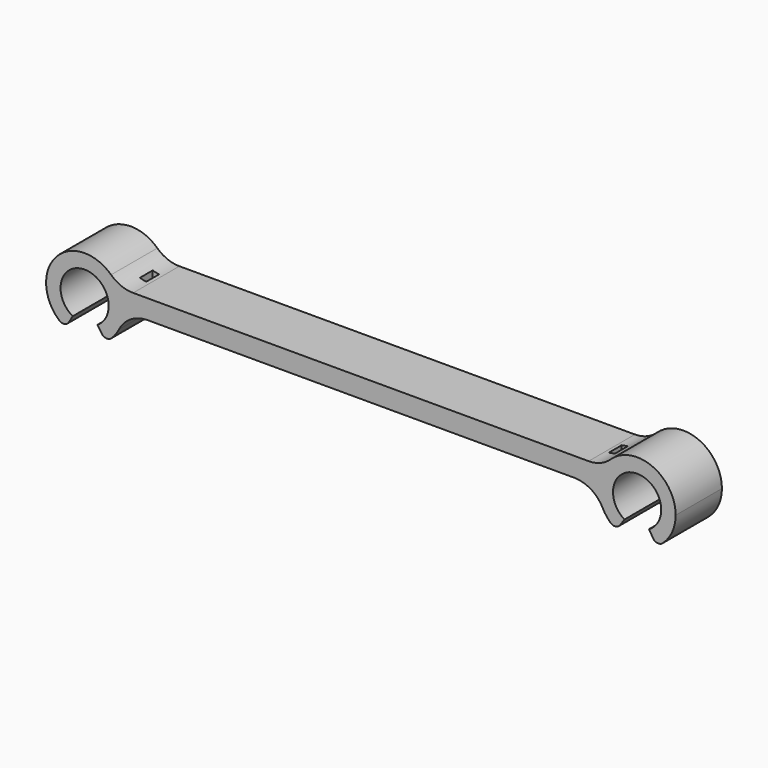
from build123d import *

# Parameters (mm, degrees)
F1_DEPTH      = 9
F2_R          = 1
F2_2_R        = 1
F3_W          = 86
F3_H          = 9
F4_DEPTH      = 3
F7_R          = 2
F8_DEPTH      = 25
F9_W          = 1
F9_H          = 2.5
F10_DEPTH     = 25
F11_R         = 3.75
F12_DEPTH     = 25
F13_T1_DEPTH  = 3.25
F13_T3_DEPTH  = 3.25
F13_T8_DEPTH  = 14.8842050314
F13_T13_DEPTH = 9
F13_T18_DEPTH = 9
F13_T23_DEPTH = 14.8842050314
F13_T28_DEPTH = 14.8842050314
F13_T33_DEPTH = 9
F13_T38_DEPTH = 9
F13_T43_DEPTH = 14.8842050314
F13_T48_DEPTH = 22.2397948557
F13_T54_DEPTH = 12.7448974278
F13_T60_DEPTH = 22.2397948557
F13_T66_DEPTH = 12.7448974278
F13_T72_DEPTH = 22.2397948557
F13_T78_DEPTH = 12.7448974278
F13_T84_DEPTH = 22.2397948557
F13_T90_DEPTH = 12.7448974278


# Not quite as in the source:
# - a fillet or chamfer that OpenCascade refuses, or shapes differently, is made with other operations: its cross-section is extruded or revolved along the edge and cut away or added
# - a feature names something its author has since deleted; it is built from what else it names


with BuildPart() as f1:
    # F0 (on Front) → F1 (new body)
    with BuildSketch(Plane.XZ):
        with BuildLine():
            ThreePointArc((-43.9727372119, -1.7475074582), (-44.0135397319, 1.7241627568), (-41, 0))
            Line((-41, 0), (-37, 0))
            ThreePointArc((-37, 0), (-46.0022354873, 5.1948611222), (-45.9955273596, -5.1987321375))
            Line((-45.9955273596, -5.1987321375), (-43.9727372119, -1.7475074582))
        make_face()
        with BuildLine():
            Line((-37, 0), (-41, 0))
            ThreePointArc((-41, 0), (-41.2758372432, -1.0135397319), (-42.0272627881, -1.7475074582))
            Line((-42.0272627881, -1.7475074582), (-39.7389427056, -5.0364179059))
            ThreePointArc((-39.7389427056, -5.0364179059), (-37.7290255281, -2.8665010233), (-37, 0))
        make_face()
    extrude(amount=F1_DEPTH)

    # F2
    f2_edges = [f1.edges().sort_by_distance(p)[0] for p in [
        (-42.027263, -4.5, -1.747507),
        (-43.972737, -4.5, -1.747507),
        (-39.738943, -4.5, -5.036418),
        (-45.995527, -4.5, -5.198732),
    ]]
    fillet(f2_edges, radius=F2_R)



with BuildPart() as f1b:
    # F0 (on Front) → F1, piece 2 (new body)
    with BuildSketch(Plane.XZ):
        with BuildLine():
            Line((41, 0), (37, 0))
            ThreePointArc((37, 0), (37.7290255281, -2.8665010233), (39.7389427056, -5.0364179059))
            Line((39.7389427056, -5.0364179059), (42.0272627881, -1.7475074582))
            ThreePointArc((42.0272627881, -1.7475074582), (41.2758372432, -1.0135397319), (41, 0))
        make_face()
        with BuildLine():
            ThreePointArc((49, 0), (43, 6), (37, 0))
            Line((37, 0), (41, 0))
            ThreePointArc((41, 0), (43, 2), (45, 0))
            ThreePointArc((45, 0), (44.7241627568, -1.0135397319), (43.9727372119, -1.7475074582))
            Line((43.9727372119, -1.7475074582), (45.9955273596, -5.1987321375))
            ThreePointArc((45.9955273596, -5.1987321375), (48.1948611222, -3.0022354873), (49, 0))
        make_face()
    extrude(amount=F1_DEPTH)

    # F2#2
    f2_2_edges = [f1b.edges().sort_by_distance(p)[0] for p in [
        (42.027263, -4.5, -1.747507),
        (43.972737, -4.5, -1.747507),
        (39.738943, -4.5, -5.036418),
        (45.995527, -4.5, -5.198732),
    ]]
    fillet(f2_2_edges, radius=F2_2_R)


with BuildPart() as f1_1:
    add(f1.part)

    add(f1b.part)  # F4 merges F1b
    # F3 (on Top) → F4 (join)
    with BuildSketch(Plane.XY):
        with Locations((0.0100198983, -4.5)):
            Rectangle(F3_W, F3_H)
    extrude(amount=F4_DEPTH)

    # F5: union 

    # F6: union 

    # F7 (on Front) → F8 (cut)
    with BuildSketch(Plane.XZ):
        with Locations((-43.0078394711, 0)):
            Circle(F7_R)
        with Locations((42.9660789669, 0)):
            Circle(F7_R)
    extrude(amount=F8_DEPTH, mode=Mode.SUBTRACT)

    # F9 (on face) → F10 (cut)
    with BuildSketch(Plane(origin=(0, 0, 0), x_dir=(1, 0, 0), z_dir=(0, 0, -1))):
        with Locations((36.5, 4.5)):
            Rectangle(F9_W, F9_H)
        with Locations((-36.5, 4.5)):
            Rectangle(F9_W, F9_H)
    extrude(amount=-F10_DEPTH, mode=Mode.SUBTRACT)

    # F11 (on Front) → F12 (cut)
    with BuildSketch(Plane.XZ):
        with Locations((-43, 0)):
            Circle(F11_R)
        with Locations((43, 0)):
            Circle(F11_R)
    extrude(amount=F12_DEPTH, mode=Mode.SUBTRACT)

    # F13: fillet of radius 5 on 6 edges, made by hand

    # F13_s2 → F13_t1 (join)
    with BuildSketch(Plane.XZ.offset(5.75)):
        with BuildLine():
            ThreePointArc((-37.655658743, -2.7272727273), (-35.8132058682, -0.7359856729), (-33.2020410289, 0))
            Line((-33.2020410289, 0), (-37, 0))
            ThreePointArc((-37, 0), (-37.1662170274, -1.4024892973), (-37.655658743, -2.7272727273))
        make_face()
        with BuildLine():
            ThreePointArc((37.655658743, -2.7272727273), (35.8132058682, -0.7359856729), (33.2020410289, 0))
            Line((33.2020410289, 0), (37, 0))
            ThreePointArc((37, 0), (37.1662170274, -1.4024892973), (37.655658743, -2.7272727273))
        make_face()
    extrude(amount=F13_T1_DEPTH)

    # F13_s4 → F13_t3 (join)
    with BuildSketch(Plane.XZ):
        with BuildLine():
            ThreePointArc((37.655658743, -2.7272727273), (35.8132058682, -0.7359856729), (33.2020410289, 0))
            Line((33.2020410289, 0), (37, 0))
            ThreePointArc((37, 0), (37.1662170274, -1.4024892973), (37.655658743, -2.7272727273))
        make_face()
        with BuildLine():
            ThreePointArc((-37.655658743, -2.7272727273), (-35.8132058682, -0.7359856729), (-33.2020410289, 0))
            Line((-33.2020410289, 0), (-37, 0))
            ThreePointArc((-37, 0), (-37.1662170274, -1.4024892973), (-37.655658743, -2.7272727273))
        make_face()
    extrude(amount=F13_T3_DEPTH)


with BuildPart() as f13_tool6:
    # F13_s7 → F13_t8 (new body)
    with BuildSketch(Plane.XZ.offset(9)):
        with BuildLine():
            ThreePointArc((35.4501655647, 3), (37.2965379294, 3.3533981136), (38.8819084899, 4.3636363636))
            ThreePointArc((38.8819084899, 4.3636363636), (38.2932324209, 3.7210669111), (37.8038475773, 3))
            Line((37.8038475773, 3), (35.4501655647, 3))
        make_face()
    extrude(amount=-F13_T8_DEPTH)

    split(bisect_by=Plane.XZ.offset(5.75), keep=Keep.TOP)


with BuildPart() as f1_2:
    add(f1_1.part)

    # F13_t5: union F13_tool6
    add(f13_tool6.part)


with BuildPart() as f13_tool11:
    # F13_s12 → F13_t13 (new body)
    with BuildSketch(Plane.XZ.offset(9)):
        with BuildLine():
            ThreePointArc((35.4501655647, 3), (37.2965379294, 3.3533981136), (38.8819084899, 4.3636363636))
            ThreePointArc((38.8819084899, 4.3636363636), (38.2932324209, 3.7210669111), (37.8038475773, 3))
            Line((37.8038475773, 3), (35.4501655647, 3))
        make_face()
    extrude(amount=-F13_T13_DEPTH)

    split(bisect_by=Plane.YZ.offset(36), keep=Keep.BOTTOM)


with BuildPart() as f1_3:
    add(f1_2.part)

    # F13_t10: union F13_tool11
    add(f13_tool11.part)


with BuildPart() as f13_tool16:
    # F13_s17 → F13_t18 (new body)
    with BuildSketch(Plane.XZ.offset(9)):
        with BuildLine():
            ThreePointArc((35.4501655647, 3), (37.2965379294, 3.3533981136), (38.8819084899, 4.3636363636))
            ThreePointArc((38.8819084899, 4.3636363636), (38.2932324209, 3.7210669111), (37.8038475773, 3))
            Line((37.8038475773, 3), (35.4501655647, 3))
        make_face()
    extrude(amount=-F13_T18_DEPTH)

    split(bisect_by=Plane.YZ.offset(37), keep=Keep.TOP)


with BuildPart() as f1_4:
    add(f1_3.part)

    # F13_t15: union F13_tool16
    add(f13_tool16.part)


with BuildPart() as f13_tool21:
    # F13_s22 → F13_t23 (new body)
    with BuildSketch(Plane.XZ.offset(14.8842050314)):
        with BuildLine():
            ThreePointArc((35.4501655647, 3), (37.2965379294, 3.3533981136), (38.8819084899, 4.3636363636))
            ThreePointArc((38.8819084899, 4.3636363636), (38.2932324209, 3.7210669111), (37.8038475773, 3))
            Line((37.8038475773, 3), (35.4501655647, 3))
        make_face()
    extrude(amount=-F13_T23_DEPTH)

    split(bisect_by=Plane.XZ.offset(3.25), keep=Keep.BOTTOM)


with BuildPart() as f1_5:
    add(f1_4.part)

    # F13_t20: union F13_tool21
    add(f13_tool21.part)


with BuildPart() as f13_tool26:
    # F13_s27 → F13_t28 (new body)
    with BuildSketch(Plane.XZ.offset(9)):
        with BuildLine():
            ThreePointArc((-35.4501655647, 3), (-37.2965379294, 3.3533981136), (-38.8819084899, 4.3636363636))
            ThreePointArc((-38.8819084899, 4.3636363636), (-38.2932324209, 3.7210669111), (-37.8038475773, 3))
            Line((-37.8038475773, 3), (-35.4501655647, 3))
        make_face()
    extrude(amount=-F13_T28_DEPTH)

    split(bisect_by=Plane.XZ.offset(5.75), keep=Keep.TOP)


with BuildPart() as f1_6:
    add(f1_5.part)

    # F13_t25: union F13_tool26
    add(f13_tool26.part)


with BuildPart() as f13_tool31:
    # F13_s32 → F13_t33 (new body)
    with BuildSketch(Plane.XZ.offset(9)):
        with BuildLine():
            ThreePointArc((-35.4501655647, 3), (-37.2965379294, 3.3533981136), (-38.8819084899, 4.3636363636))
            ThreePointArc((-38.8819084899, 4.3636363636), (-38.2932324209, 3.7210669111), (-37.8038475773, 3))
            Line((-37.8038475773, 3), (-35.4501655647, 3))
        make_face()
    extrude(amount=-F13_T33_DEPTH)

    split(bisect_by=Plane.YZ.offset(-36), keep=Keep.TOP)


with BuildPart() as f1_7:
    add(f1_6.part)

    # F13_t30: union F13_tool31
    add(f13_tool31.part)


with BuildPart() as f13_tool36:
    # F13_s37 → F13_t38 (new body)
    with BuildSketch(Plane.XZ.offset(9)):
        with BuildLine():
            ThreePointArc((-35.4501655647, 3), (-37.2965379294, 3.3533981136), (-38.8819084899, 4.3636363636))
            ThreePointArc((-38.8819084899, 4.3636363636), (-38.2932324209, 3.7210669111), (-37.8038475773, 3))
            Line((-37.8038475773, 3), (-35.4501655647, 3))
        make_face()
    extrude(amount=-F13_T38_DEPTH)

    split(bisect_by=Plane.YZ.offset(-37), keep=Keep.BOTTOM)


with BuildPart() as f1_8:
    add(f1_7.part)

    # F13_t35: union F13_tool36
    add(f13_tool36.part)


with BuildPart() as f13_tool41:
    # F13_s42 → F13_t43 (new body)
    with BuildSketch(Plane.XZ.offset(14.8842050314)):
        with BuildLine():
            ThreePointArc((-35.4501655647, 3), (-37.2965379294, 3.3533981136), (-38.8819084899, 4.3636363636))
            ThreePointArc((-38.8819084899, 4.3636363636), (-38.2932324209, 3.7210669111), (-37.8038475773, 3))
            Line((-37.8038475773, 3), (-35.4501655647, 3))
        make_face()
    extrude(amount=-F13_T43_DEPTH)

    split(bisect_by=Plane.XZ.offset(3.25), keep=Keep.BOTTOM)


with BuildPart() as f1_9:
    add(f1_8.part)

    # F13_t40: union F13_tool41
    add(f13_tool41.part)


with BuildPart() as f13_tool46:
    # F13_s47 → F13_t48 (new body)
    with BuildSketch(Plane.XZ.offset(18.4948974278)):
        with BuildLine():
            ThreePointArc((-37.655658743, -2.7272727273), (-35.8132058682, -0.7359856729), (-33.2020410289, 0))
            Line((-33.2020410289, 0), (-37, 0))
            ThreePointArc((-37, 0), (-37.1662170274, -1.4024892973), (-37.655658743, -2.7272727273))
        make_face()
    extrude(amount=-F13_T48_DEPTH)

    split(bisect_by=Plane.XZ.offset(3.25), keep=Keep.BOTTOM)

    split(bisect_by=Plane.XZ, keep=Keep.TOP)


with BuildPart() as f1_10:
    add(f1_9.part)

    # F13_t45: union F13_tool46
    add(f13_tool46.part)


with BuildPart() as f13_tool52:
    # F13_s53 → F13_t54 (new body)
    with BuildSketch(Plane.XZ.offset(9)):
        with BuildLine():
            ThreePointArc((-37.655658743, -2.7272727273), (-35.8132058682, -0.7359856729), (-33.2020410289, 0))
            Line((-33.2020410289, 0), (-37, 0))
            ThreePointArc((-37, 0), (-37.1662170274, -1.4024892973), (-37.655658743, -2.7272727273))
        make_face()
    extrude(amount=-F13_T54_DEPTH)

    split(bisect_by=Plane.YZ.offset(-36), keep=Keep.TOP)

    split(bisect_by=Plane.XZ, keep=Keep.TOP)


with BuildPart() as f1_11:
    add(f1_10.part)

    # F13_t51: union F13_tool52
    add(f13_tool52.part)


with BuildPart() as f13_tool58:
    # F13_s59 → F13_t60 (new body)
    with BuildSketch(Plane.XZ.offset(18.4948974278)):
        with BuildLine():
            ThreePointArc((37.655658743, -2.7272727273), (35.8132058682, -0.7359856729), (33.2020410289, 0))
            Line((33.2020410289, 0), (37, 0))
            ThreePointArc((37, 0), (37.1662170274, -1.4024892973), (37.655658743, -2.7272727273))
        make_face()
    extrude(amount=-F13_T60_DEPTH)

    split(bisect_by=Plane.XZ.offset(3.25), keep=Keep.BOTTOM)

    split(bisect_by=Plane.XZ, keep=Keep.TOP)


with BuildPart() as f1_12:
    add(f1_11.part)

    # F13_t57: union F13_tool58
    add(f13_tool58.part)


with BuildPart() as f13_tool64:
    # F13_s65 → F13_t66 (new body)
    with BuildSketch(Plane.XZ.offset(9)):
        with BuildLine():
            ThreePointArc((37.655658743, -2.7272727273), (35.8132058682, -0.7359856729), (33.2020410289, 0))
            Line((33.2020410289, 0), (37, 0))
            ThreePointArc((37, 0), (37.1662170274, -1.4024892973), (37.655658743, -2.7272727273))
        make_face()
    extrude(amount=-F13_T66_DEPTH)

    split(bisect_by=Plane.YZ.offset(36), keep=Keep.BOTTOM)

    split(bisect_by=Plane.XZ, keep=Keep.TOP)


with BuildPart() as f1_13:
    add(f1_12.part)

    # F13_t63: union F13_tool64
    add(f13_tool64.part)


with BuildPart() as f13_tool70:
    # F13_s71 → F13_t72 (new body)
    with BuildSketch(Plane.XZ.offset(12.7448974278)):
        with BuildLine():
            ThreePointArc((37.655658743, -2.7272727273), (35.8132058682, -0.7359856729), (33.2020410289, 0))
            Line((33.2020410289, 0), (37, 0))
            ThreePointArc((37, 0), (37.1662170274, -1.4024892973), (37.655658743, -2.7272727273))
        make_face()
    extrude(amount=-F13_T72_DEPTH)

    split(bisect_by=Plane.XZ.offset(5.75), keep=Keep.TOP)

    split(bisect_by=Plane.XZ.offset(9), keep=Keep.BOTTOM)


with BuildPart() as f1_14:
    add(f1_13.part)

    # F13_t69: union F13_tool70
    add(f13_tool70.part)


with BuildPart() as f13_tool76:
    # F13_s77 → F13_t78 (new body)
    with BuildSketch(Plane.XZ.offset(12.7448974278)):
        with BuildLine():
            ThreePointArc((37.655658743, -2.7272727273), (35.8132058682, -0.7359856729), (33.2020410289, 0))
            Line((33.2020410289, 0), (37, 0))
            ThreePointArc((37, 0), (37.1662170274, -1.4024892973), (37.655658743, -2.7272727273))
        make_face()
    extrude(amount=-F13_T78_DEPTH)

    split(bisect_by=Plane.YZ.offset(36), keep=Keep.BOTTOM)

    split(bisect_by=Plane.XZ.offset(9), keep=Keep.BOTTOM)


with BuildPart() as f1_15:
    add(f1_14.part)

    # F13_t75: union F13_tool76
    add(f13_tool76.part)


with BuildPart() as f13_tool82:
    # F13_s83 → F13_t84 (new body)
    with BuildSketch(Plane.XZ.offset(12.7448974278)):
        with BuildLine():
            ThreePointArc((-37.655658743, -2.7272727273), (-35.8132058682, -0.7359856729), (-33.2020410289, 0))
            Line((-33.2020410289, 0), (-37, 0))
            ThreePointArc((-37, 0), (-37.1662170274, -1.4024892973), (-37.655658743, -2.7272727273))
        make_face()
    extrude(amount=-F13_T84_DEPTH)

    split(bisect_by=Plane.XZ.offset(5.75), keep=Keep.TOP)

    split(bisect_by=Plane.XZ.offset(9), keep=Keep.BOTTOM)


with BuildPart() as f1_16:
    add(f1_15.part)

    # F13_t81: union F13_tool82
    add(f13_tool82.part)


with BuildPart() as f13_tool88:
    # F13_s89 → F13_t90 (new body)
    with BuildSketch(Plane.XZ.offset(12.7448974278)):
        with BuildLine():
            ThreePointArc((-37.655658743, -2.7272727273), (-35.8132058682, -0.7359856729), (-33.2020410289, 0))
            Line((-33.2020410289, 0), (-37, 0))
            ThreePointArc((-37, 0), (-37.1662170274, -1.4024892973), (-37.655658743, -2.7272727273))
        make_face()
    extrude(amount=-F13_T90_DEPTH)

    split(bisect_by=Plane.YZ.offset(-36), keep=Keep.TOP)

    split(bisect_by=Plane.XZ.offset(9), keep=Keep.BOTTOM)


with BuildPart() as f1_17:
    add(f1_16.part)

    # F13_t87: union F13_tool88
    add(f13_tool88.part)


solid = f1_17.part
